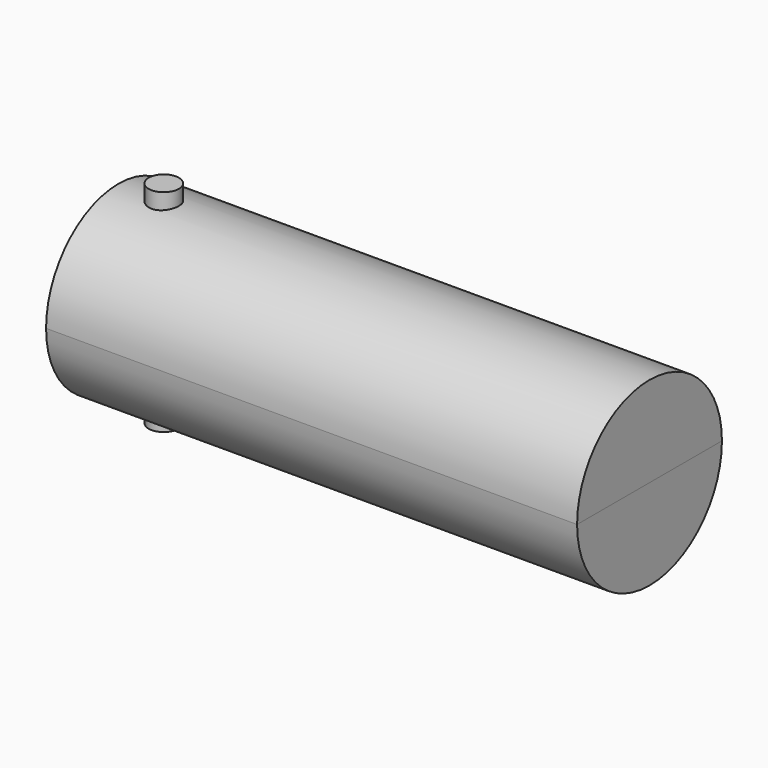
from build123d import *
from build123d import SkipClean  # not in build123d's __all__

# Parameters (mm, degrees)
F1_DEPTH = 8.8
F2_R     = 0.25
F3_DEPTH = 1.75


with BuildPart() as f1:
    # F0 (on Right) → F1 (new body)
    with BuildSketch(Plane.YZ):
        with BuildLine():
            Line((-1.5, 0), (1.5, 0))
            ThreePointArc((1.5, 0), (0, 1.5), (-1.5, 0))
        make_face()
    extrude(amount=F1_DEPTH)

    # F2 (on face) → F3 (join, symmetric)
    with BuildSketch(Plane(origin=(0, 0, 0), x_dir=(1, 0, 0), z_dir=(0, 0, -1))):
        with Locations((0.75, 0)):
            Circle(F2_R)
    extrude(amount=F3_DEPTH, both=True)

    # F4: F1 across plane


with BuildPart() as f1_1:
    add(f1.part, clean=False)
    with SkipClean():  # cleaning this boolean's faces spoils the solid; the shape is the same uncleaned
        add(f1.part.mirror(Plane.XY), clean=False)


solid = f1_1.part
